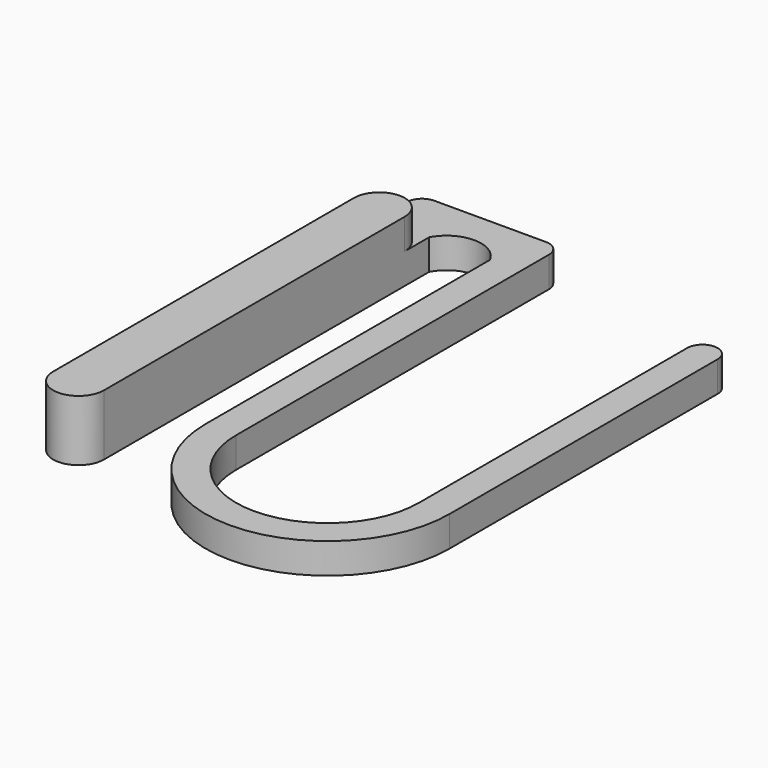
from build123d import *

# Parameters (mm, degrees)
F1_DEPTH = 3
F3_DEPTH = 3
F4_R     = 1.5


with BuildPart() as f1:
    # F0 (on Top) → F1 (new body)
    with BuildSketch(Plane.XY):
        with BuildLine():
            ThreePointArc((9, 0), (0, -9), (-9, 0))
            Line((-9, 0), (-9, 40))
            Line((-9, 40), (-23, 40))
            Line((-23, 40), (-23, -5))
            ThreePointArc((-23, -5), (-20.5, -7.5), (-18, -5))
            Line((-18, -5), (-18, 35))
            ThreePointArc((-18, 35), (-15, 36.8), (-12, 35))
            Line((-12, 35), (-12, 0))
            ThreePointArc((-12, 0), (0, -12), (12, 0))
            Line((12, 0), (12, 33))
            ThreePointArc((12, 33), (10.5, 34.5), (9, 33))
            Line((9, 33), (9, 0))
        make_face()
    extrude(amount=F1_DEPTH)

    # F2 (on face) → F3 (join)
    with BuildSketch(Plane.XY.offset(3)):
        with BuildLine():
            Line((-18, -5), (-18, 32))
            ThreePointArc((-18, 32), (-20.5, 34.5), (-23, 32))
            Line((-23, 32), (-23, -5))
            ThreePointArc((-23, -5), (-20.5, -7.5), (-18, -5))
        make_face()
    extrude(amount=F3_DEPTH)

    # F4
    f4_edges = [f1.edges().sort_by_distance(p)[0] for p in [
        (-23, 40, 1.5),
        (-9, 40, 1.5),
    ]]
    fillet(f4_edges, radius=F4_R)


solid = f1.part
